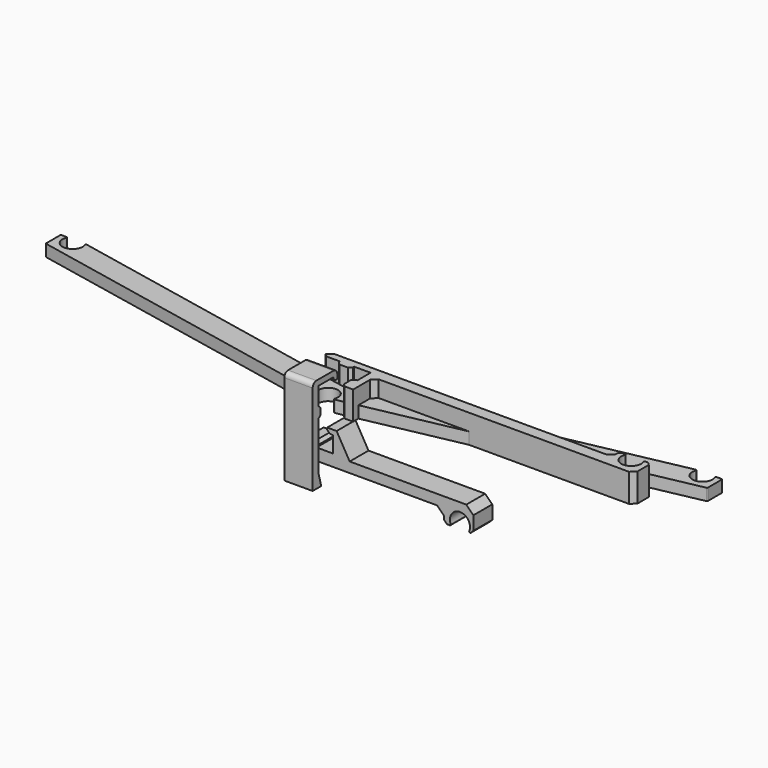
from build123d import *

# Parameters (mm, degrees)
F2_DEPTH    = 10
F3_SIZE     = 1.2
F4_SIZE     = 3
F6_DEPTH    = 12
F7_SIZE     = 1.2
F8_T1_DEPTH = 12
F8_T3_DEPTH = 22.2867319519
F9_R        = 0.4
F9_2_R      = 0.4
F15_DEPTH   = 5
F16_R       = 0.4
F12_DEPTH   = 12
F13_SIZE    = 0.8
F14_R       = 2


# Not quite as in the source:
# - a fillet or chamfer that OpenCascade refuses, or shapes differently, is made with other operations: its cross-section is extruded or revolved along the edge and cut away or added


with BuildPart() as f2:
    # F1 (on Front) → F2 (new body)
    with BuildSketch(Plane.XZ):
        with BuildLine():
            Line((7.6, -1.1), (7.6, -3.1))
            Line((7.6, -3.1), (10, -3.1))
            Line((10, -3.1), (10, -10))
            Line((10, -10), (3.1, -10))
            Line((3.1, -10), (3.1, -8.2))
            Line((3.1, -8.2), (-3.1, -8.2))
            Line((-3.1, -8.2), (-3.1, -10))
            Line((-3.1, -10), (-9, -10))
            Line((-9, -10), (-9, -15))
            Line((-9, -15), (57.2193920339, -15))
            Line((57.2193920339, -15), (57.2193920339, -20.675))
            Line((57.2193920339, -20.675), (60.2193920339, -20.675))
            ThreePointArc((60.2193920339, -20.675), (62.8000190583, -14.4448152383), (68.15, -18.55))
            ThreePointArc((68.15, -18.55), (68.0051847617, -19.6499809417), (67.5806079661, -20.675))
            Line((67.5806079661, -20.675), (69.5806079661, -20.675))
            Line((69.5806079661, -20.675), (69.5806079661, -10.675))
            Line((69.5806079661, -10.675), (17.1281288275, -10.675))
            Line((17.1281288275, -10.675), (11.6, -1.1))
            Line((11.6, -1.1), (7.6, -1.1))
        make_face()
    extrude(amount=F2_DEPTH)

    # F3
    f3_edges = [f2.edges().sort_by_distance(p)[0] for p in [
        (-3.1, -5, -8.2),
        (3.1, -5, -8.2),
        (7.6, -5, -3.1),
        (57.219392, -5, -20.675),
        (69.580608, -5, -20.675),
    ]]
    chamfer(f3_edges, length=F3_SIZE)

    # F4
    f4_edges = [f2.edges().sort_by_distance(p)[0] for p in [
        (-9, -5, -15),
        (57.219392, -5, -15),
        (69.580608, -5, -10.675),
    ]]
    chamfer(f4_edges, length=F4_SIZE)

    # F9
    f9_edges = [f2.edges().sort_by_distance(p)[0] for p in [
        (60.219392, -5, -20.675),
        (67.580608, -5, -20.675),
    ]]
    fillet(f9_edges, radius=F9_R)


with BuildPart() as f6:
    # F5 (on Top) → F6 (new body)
    with BuildSketch(Plane.XY):
        with BuildLine():
            ThreePointArc((120.1806079661, 17.125), (120.6051847617, 16.0999809417), (120.75, 15))
            ThreePointArc((120.75, 15), (115.4000190583, 10.8948152383), (112.8193920339, 17.125))
            Line((112.8193920339, 17.125), (109.8193920339, 17.125))
            Line((109.8193920339, 17.125), (109.8193920339, 13))
            Line((109.8193920339, 13), (-10, 13))
            Line((-10, 13), (-10, 10))
            Line((-10, 10), (-3, 10))
            Line((-3, 10), (-3, 8.2))
            Line((-3, 8.2), (3, 8.2))
            Line((3, 8.2), (3, 10))
            Line((3, 10), (10, 10))
            Line((10, 10), (10, 3))
            Line((10, 3), (8.2, 3))
            Line((8.2, 3), (8.2, -3))
            Line((8.2, -3), (10, -3))
            Line((10, -3), (13, -3))
            Line((13, -3), (13, 8))
            Line((13, 8), (123.1806079661, 8))
            Line((123.1806079661, 8), (123.1806079661, 17.125))
            Line((123.1806079661, 17.125), (120.1806079661, 17.125))
        make_face()
    extrude(amount=F6_DEPTH)

    # F7
    f7_edges = [f6.edges().sort_by_distance(p)[0] for p in [
        (8.2, 3, 6),
        (8.2, -3, 6),
        (-3, 8.2, 6),
        (3, 8.2, 6),
        (-10, 10, 6),
        (109.819392, 17.125, 6),
        (123.180608, 17.125, 6),
    ]]
    chamfer(f7_edges, length=F7_SIZE)

    # F8: chamfer of 2 on 4 edges, made by hand

    # F8_s2 → F8_t1 (join)
    with BuildSketch(Plane.XY):
        Polygon((15, 8), (13, 6), (13, 8), align=None)
        Polygon((109.8193920339, 15), (107.8193920339, 13), (109.8193920339, 13), align=None)
    extrude(amount=F8_T1_DEPTH)

    # F8_s4 → F8_t3 (cut)
    with BuildSketch(Plane.XY.offset(-5.1433659759)):
        Polygon((-8, 13), (-10, 11), (-10, 13), align=None)
        Polygon((123.1806079661, 10), (121.1806079661, 8), (123.1806079661, 8), align=None)
    extrude(amount=F8_T3_DEPTH, mode=Mode.SUBTRACT)

    # F9#2
    f9_2_edges = [f6.edges().sort_by_distance(p)[0] for p in [
        (112.819392, 17.125, 6),
        (120.180608, 17.125, 6),
    ]]
    fillet(f9_2_edges, radius=F9_2_R)


with BuildPart() as f15:
    # F10 (on Top) → F15 (new body)
    with BuildSketch(Plane.XY):
        with BuildLine():
            ThreePointArc((-3.6373066959, -2.1), (-1.0870399894, 4.0568884704), (4.2, 0))
            ThreePointArc((4.2, 0), (4.0568884704, -1.0870399894), (3.6373066959, -2.1))
            Line((3.6373066959, -2.1), (140.2239092363, 25.65))
            Line((140.2239092363, 25.65), (140.2239092363, 33.65))
            Line((140.2239092363, 33.65), (137.2239092363, 33.65))
            ThreePointArc((137.2239092363, 33.65), (137.653481053, 32.6129218939), (137.8, 31.5))
            ThreePointArc((137.8, 31.5), (132.3870781061, 27.346518947), (129.7760907637, 33.65))
            Line((129.7760907637, 33.65), (0, 7.2836767171))
            Line((0, 7.2836767171), (-129.7760907637, 33.65))
            ThreePointArc((-129.7760907637, 33.65), (-129.346518947, 32.6129218939), (-129.2, 31.5))
            ThreePointArc((-129.2, 31.5), (-134.6129218939, 27.346518947), (-137.2239092363, 33.65))
            Line((-137.2239092363, 33.65), (-140.2239092363, 33.65))
            Line((-140.2239092363, 33.65), (-140.2239092363, 25.65))
            Line((-140.2239092363, 25.65), (-3.6373066959, -2.1))
        make_face()
    extrude(amount=F15_DEPTH)

    # F16
    f16_edges = [f15.edges().sort_by_distance(p)[0] for p in [
        (-3.637307, -2.1, 2.5),
        (3.637307, -2.1, 2.5),
        (0, 7.283677, 2.5),
        (129.776091, 33.65, 2.5),
        (137.223909, 33.65, 2.5),
        (140.223909, 33.65, 2.5),
        (140.223909, 25.65, 2.5),
        (-140.223909, 33.65, 2.5),
        (-140.223909, 25.65, 2.5),
        (-129.776091, 33.65, 2.5),
        (-137.223909, 33.65, 2.5),
    ]]
    fillet(f16_edges, radius=F16_R)


with BuildPart() as f12:
    # F11 (on Right) → F12 (new body)
    with BuildSketch(Plane.YZ):
        Polygon((-12.15, 20), (-12.15, 18.5), (-10.15, 18.5), (-10.15, 22.4), (-23.2, 22.4), (-23.2, -18), (-18.6602540378, -18), (-20, -13), (-20, 7.85), (-19, 7.85), (-19, 12.15), (-20, 12.15), (-20, 20), align=None)
    extrude(amount=F12_DEPTH)

    # F13
    f13_edges = [f12.edges().sort_by_distance(p)[0] for p in [
        (6, -19, 12.15),
        (6, -12.15, 18.5),
        (6, -19, 7.85),
    ]]
    chamfer(f13_edges, length=F13_SIZE)

    # F14
    f14_edges = [f12.edges().sort_by_distance(p)[0] for p in [
        (6, -23.2, 22.4),
        (6, -20, -13),
        (6, -10.15, 22.4),
    ]]
    fillet(f14_edges, radius=F14_R)


solid = Compound([f2.part, f6.part, f15.part, f12.part])
